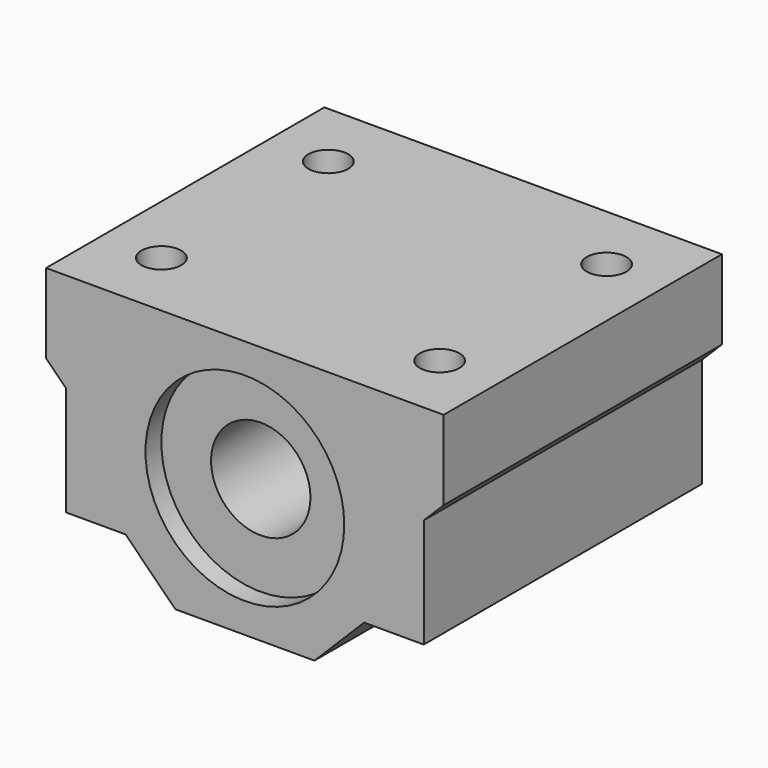
from build123d import *

# Parameters (mm, degrees)
F0_R     = 5
F1_DEPTH = 17.5
F2_R     = 10
F3_DEPTH = 2
F4_R     = 2
F5_DEPTH = 25


# Not quite as in the source:
# - a pattern or mirror of a feature is missing from the dataset's text; its kind, count and spacing are read off the source's solid


with BuildPart() as f1:
    # F0 (on Front) → F1 (new body, symmetric)
    with BuildSketch(Plane.XZ):
        Polygon((20, 13), (0, 13), (-20, 13), (-20, 5), (-18, 3), (-18, -8), (-12, -8), (-7, -13), (0, -13), (7, -13), (12, -8), (18, -8), (18, 3), (20, 5), align=None)
        Circle(F0_R, mode=Mode.SUBTRACT)
    extrude(amount=F1_DEPTH, both=True)

    # F2 (on face) → F3 (cut)
    with BuildSketch(Plane.XZ.offset(17.5)):
        Circle(F2_R)
    f3 = extrude(amount=-F3_DEPTH, mode=Mode.SUBTRACT)

    # F3_copies: F3 across plane
    add(f3.mirror(Plane.ZX), mode=Mode.SUBTRACT)

    # F4 (on face) → F5 (cut)
    with BuildSketch(Plane.XY.offset(13)):
        with Locations((-14, 10.5)):
            Circle(F4_R)
        with Locations((-14, -10.5)):
            Circle(F4_R)
        with Locations((14, 10.5)):
            Circle(F4_R)
        with Locations((14, -10.5)):
            Circle(F4_R)
    extrude(amount=-F5_DEPTH, mode=Mode.SUBTRACT)


solid = f1.part
